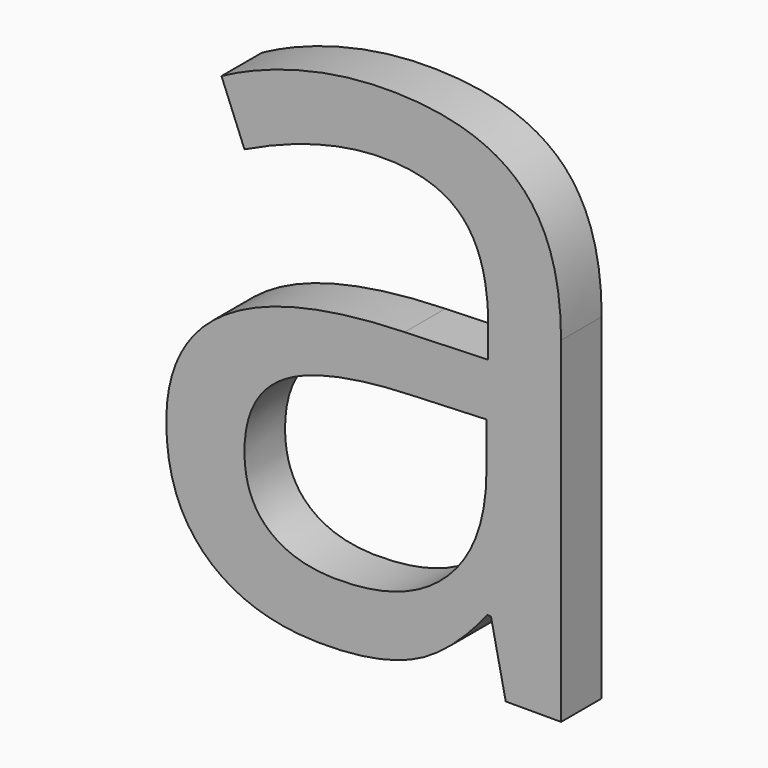
from build123d import *

# Parameters (mm, degrees)
F0_TEXT_SIZE = 46.0193233771
F1_DEPTH     = 2.54


# Not quite as in the source:
# - Text() gives the source's letters only with a copy of the font that has no kerning and outlines rounded to 1/6400 em; it was checked with that copy


with BuildPart() as f1:
    # F0 (on Front) → F1 (new body)
    with BuildSketch(Plane.XZ):
        with Locations((-24.8504346237, 0)):
            Text('a', F0_TEXT_SIZE, font='Open Sans', text_align=(TextAlign.LEFT, TextAlign.BOTTOM))
    extrude(amount=F1_DEPTH)


solid = f1.part
